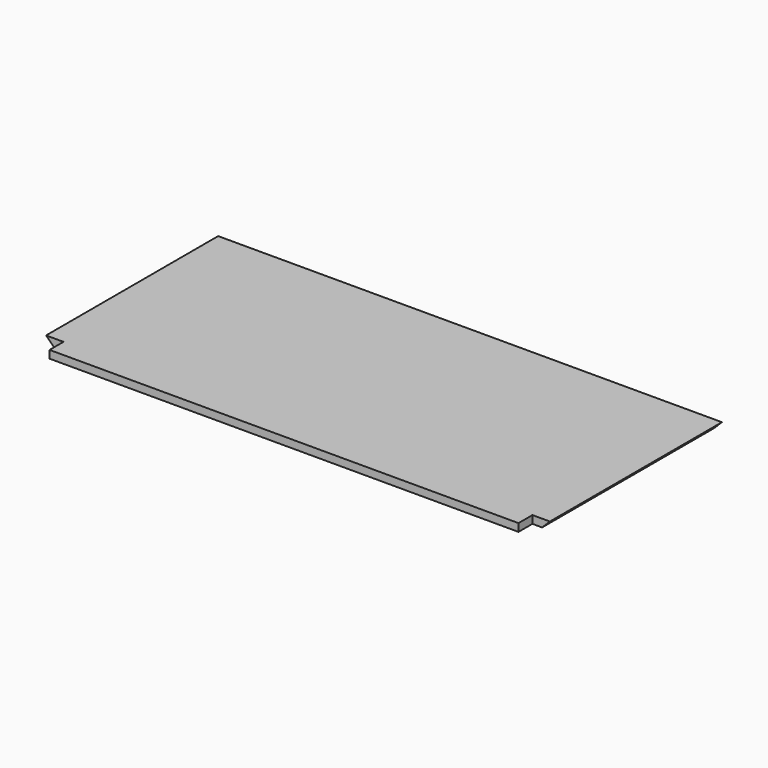
from build123d import *

# Parameters (mm, degrees)
F1_DEPTH = 20
F2_SIZE  = 19.99999


# Not quite as in the source:
# - a fillet or chamfer is up to 0.001 mm smaller than in the source, because OpenCascade refuses the exact size


with BuildPart() as f1:
    # F0 (on Top) → F1 (new body)
    with BuildSketch(Plane.XY):
        Polygon((54.2228519917, 569.4585297257), (-1245.7771480083, 569.4585297257), (-1245.7771480083, 14.4585297257), (-1200.7771480083, 14.4585297257), (-1200.7771480083, -30.5414702743), (9.2228519917, -30.5414702743), (9.2228519917, 14.4585297257), (54.2228519917, 14.4585297257), align=None)
    extrude(amount=-F1_DEPTH)

    # F2 (size 20 in the source; OpenCascade refuses exactly that, so slightly less here)
    f2_edges = [f1.edges().sort_by_distance(p)[0] for p in [
        (-1245.777148, 291.95853, -20),
        (54.222852, 291.95853, -20),
    ]]
    chamfer(f2_edges, length=F2_SIZE)


solid = f1.part
